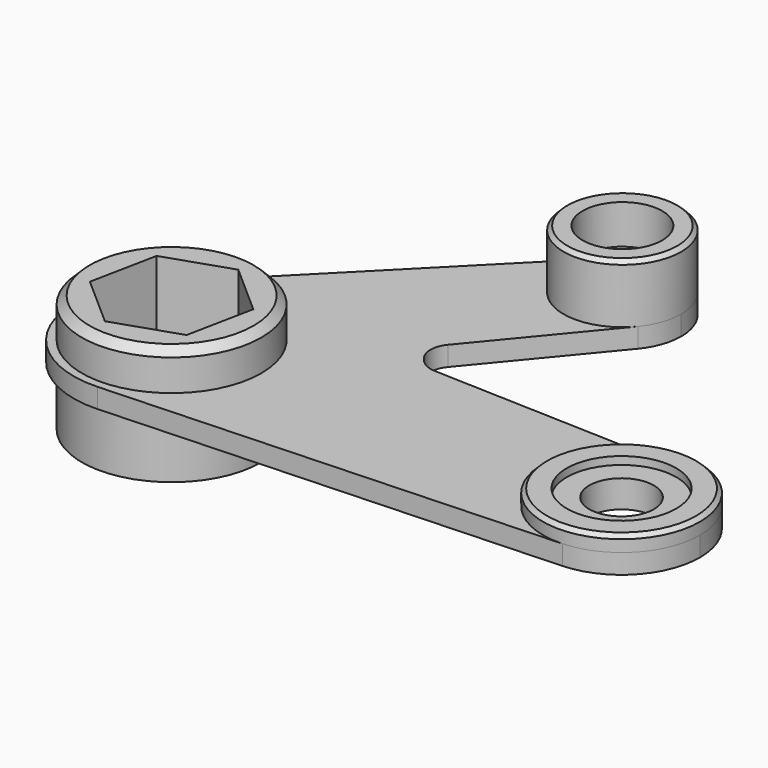
from build123d import *

# Parameters (mm, degrees)
F1_DEPTH      = 12.7
F2_R          = 58.196986
F3_DEPTH      = 25.4
F3_DEPTH_BACK = 50.8
F4_SIZE       = 5.08
F6_DEPTH      = 76.201
F7_R          = 38.1
F8_DEPTH      = 38.1
F9_SIZE       = 2.54
F10_R         = 25.791383
F11_DEPTH     = 25.4
F12_R         = 15.98943
F13_DEPTH     = 63.501
F14_R         = 50.8
F15_DEPTH     = 10.16
F16_SIZE      = 2.54
F17_R         = 35.469376
F18_DEPTH     = 5.08
F19_R         = 20.916233
F20_DEPTH     = 55.881
F21_R         = 15.24


with BuildPart() as f1:
    # F0 (on Top) → F1 (new body)
    with BuildSketch(Plane.XY):
        with BuildLine():
            ThreePointArc((-101.565805, -63.439695), (-58.463537, -43.912178), (-40.832597, 0))
            ThreePointArc((-40.832597, 0), (-80.185359, 58.729557), (-149.467586, 44.666349))
            ThreePointArc((-149.467586, 44.666349), (-162.388563, -25.724595), (-101.565805, -63.439695))
        make_face()
        with BuildLine():
            ThreePointArc((-149.467586, 44.666349), (-80.185359, 58.729557), (-40.832597, 0))
            ThreePointArc((-40.832597, 0), (-58.463537, -43.912178), (-101.565805, -63.439695))
            Line((-101.565805, -63.439695), (189.355582, -50.751756))
            ThreePointArc((189.355582, -50.751756), (136.342602, -0.214732), (188.926451, 50.768654))
            Line((188.926451, 50.768654), (13.851842, 56.921783))
            Line((13.851842, 56.921783), (0, 73.46686))
            Line((0, 73.46686), (70.550478, 158.881204))
            ThreePointArc((70.550478, 158.881204), (15.61797, 154.887936), (14.094289, 209.944317))
            Line((14.094289, 209.944317), (-149.467586, 44.666349))
        make_face()
        with BuildLine():
            ThreePointArc((79.275282, 183.144507), (55.663625, 218.382242), (14.094289, 209.944317))
            ThreePointArc((14.094289, 209.944317), (15.61797, 154.887936), (70.550478, 158.881204))
            ThreePointArc((70.550478, 158.881204), (77.027792, 170.252358), (79.275282, 183.144507))
        make_face()
        with BuildLine():
            ThreePointArc((188.926451, 50.768654), (136.342602, -0.214732), (189.355582, -50.751756))
            ThreePointArc((189.355582, -50.751756), (223.837396, -35.129742), (237.942149, 0))
            ThreePointArc((237.942149, 0), (223.688575, 35.284539), (188.926451, 50.768654))
        make_face()
    extrude(amount=F1_DEPTH)

    # F2 (on face) → F3 (join, two sides)
    with BuildSketch(Plane.XY.offset(12.7)) as f3_sk:
        with Locations((-104.332597, 0)):
            Circle(F2_R)
    extrude(amount=F3_DEPTH)
    extrude(f3_sk.sketch, amount=-F3_DEPTH_BACK)

    # F4
    f4_edges = [f1.edges().sort_by_distance(p)[0] for p in [
        (-162.529583, 0, 38.1),
    ]]
    chamfer(f4_edges, length=F4_SIZE)

    # F5 (on face) → F6 (cut, through all)
    with BuildSketch(Plane.XY.offset(38.1)):
        Polygon((-113.029572, -43.125893), (-71.332966, -29.094748), (-62.635991, 14.031145), (-95.635622, 43.125893), (-137.332228, 29.094748), (-146.029203, -14.031145), align=None)
    extrude(amount=-F6_DEPTH, mode=Mode.SUBTRACT)

    # F7 (on face) → F8 (join)
    with BuildSketch(Plane.XY.offset(12.7)):
        with Locations((41.175282, 183.144507)):
            Circle(F7_R)
    extrude(amount=F8_DEPTH)

    # F9
    f9_edges = [f1.edges().sort_by_distance(p)[0] for p in [
        (3.075282, 183.144507, 50.8),
    ]]
    chamfer(f9_edges, length=F9_SIZE)

    # F10 (on face) → F11 (cut)
    with BuildSketch(Plane.XY.offset(50.8)):
        with Locations((41.175282, 183.144507)):
            Circle(F10_R)
    extrude(amount=-F11_DEPTH, mode=Mode.SUBTRACT)

    # F12 (on face) → F13 (cut, through all)
    with BuildSketch(Plane.XY.offset(25.4)):
        with Locations((41.175282, 183.144507)):
            Circle(F12_R)
    extrude(amount=-F13_DEPTH, mode=Mode.SUBTRACT)

    # F14 (on face) → F15 (join)
    with BuildSketch(Plane.XY.offset(12.7)):
        with Locations((187.142149, 0)):
            Circle(F14_R)
    extrude(amount=F15_DEPTH)

    # F16
    f16_edges = [f1.edges().sort_by_distance(p)[0] for p in [
        (136.342149, 0, 22.86),
    ]]
    chamfer(f16_edges, length=F16_SIZE)

    # F17 (on face) → F18 (cut)
    with BuildSketch(Plane.XY.offset(22.86)):
        with Locations((187.142149, 0)):
            Circle(F17_R)
    extrude(amount=-F18_DEPTH, mode=Mode.SUBTRACT)

    # F19 (on face) → F20 (cut, through all)
    with BuildSketch(Plane.XY.offset(17.78)):
        with Locations((187.142149, 0)):
            Circle(F19_R)
    extrude(amount=-F20_DEPTH, mode=Mode.SUBTRACT)

    # F21
    f21_edges = [f1.edges().sort_by_distance(p)[0] for p in [
        (0, 73.46686, 6.35),
        (13.851842, 56.921783, 6.35),
    ]]
    fillet(f21_edges, radius=F21_R)


solid = f1.part
